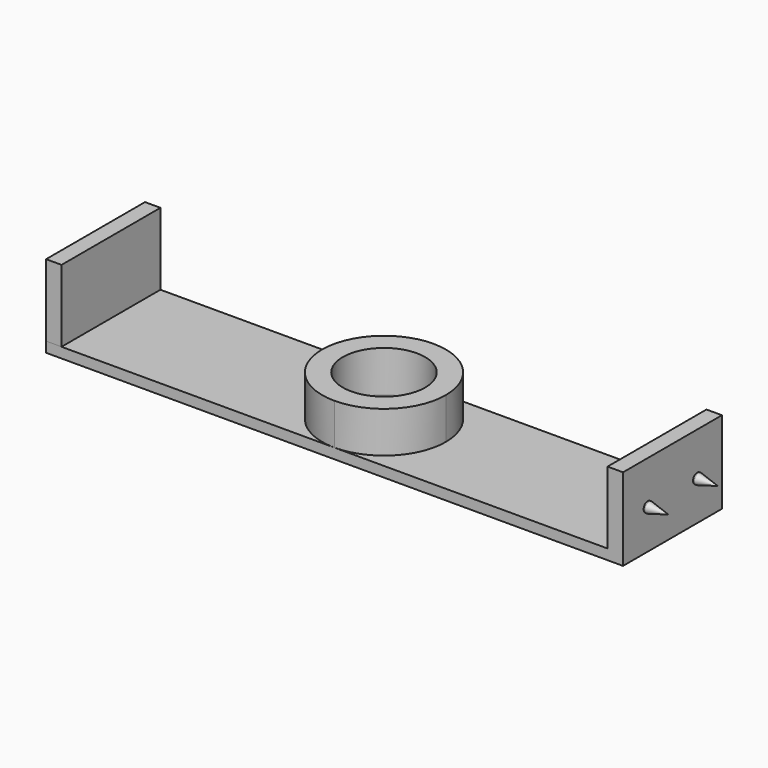
from build123d import *

# Parameters (mm, degrees)
F0_W        = 56
F0_H        = 12
F1_DEPTH    = 1
F2_W        = 12
F2_H        = 12
F2_R        = 4
F3_DEPTH    = 4
F4_DEPTH    = 25
F5_R        = 5.99999
F6_W        = 12
F6_H        = 7
F7_DEPTH    = 1.5
F8_W        = 12
F8_H        = 7
F9_DEPTH    = 1.5
F10_R       = 0.5
F11_DEPTH   = 2
F12_R       = 0.5
F13_DEPTH   = 2
F14_SIZE2   = 1.8660254038
F14_SIZE    = 0.5
F14_2_SIZE2 = 1.8660254038
F14_2_SIZE  = 0.5
F14_3_SIZE2 = 1.8660254038
F14_3_SIZE  = 0.5
F14_4_SIZE2 = 1.8660254038
F14_4_SIZE  = 0.5


# Not quite as in the source:
# - a fillet or chamfer is up to 0.001 mm smaller than in the source, because OpenCascade refuses the exact size


with BuildPart() as f1:
    # F0 (on Top) → F1 (new body)
    with BuildSketch(Plane.XY):
        Rectangle(F0_W, F0_H)
    extrude(amount=F1_DEPTH)

    # F2 (on face) → F3 (join)
    with BuildSketch(Plane.XY.offset(1)):
        Rectangle(F2_W, F2_H)
        Circle(F2_R, mode=Mode.SUBTRACT)
    extrude(amount=F3_DEPTH)

    # F4 (cut): a face of the model
    f4_faces = [f1.faces().sort_by_distance(p)[0] for p in [
        (0, 0, 1),
    ]]
    extrude(f4_faces, amount=-F4_DEPTH, mode=Mode.SUBTRACT)

    # F5 (radius 6 in the source; OpenCascade refuses exactly that, so slightly less here)
    f5_edges = [f1.edges().sort_by_distance(p)[0] for p in [
        (6, 6, 3),
        (6, -6, 3),
        (-6, -6, 3),
        (-6, 6, 3),
    ]]
    fillet(f5_edges, radius=F5_R)

    # F6 (on face) → F7 (join)
    with BuildSketch(Plane.YZ.offset(28)):
        with Locations((0, 4.5)):
            Rectangle(F6_W, F6_H)
    extrude(amount=-F7_DEPTH)

    # F10 (on face) → F11 (join)
    with BuildSketch(Plane.YZ.offset(28)):
        with Locations((3, 3.8193718065)):
            Circle(F10_R)
        with Locations((-3, 3.8193718065)):
            Circle(F10_R)
    extrude(amount=F11_DEPTH)

    # F14
    f14_edges = [f1.edges().sort_by_distance(p)[0] for p in [
        (30, 2.5, 3.819372),
    ]]
    f14_side = f1.faces().sort_by_distance((30, 3, 3.819372))[0]
    chamfer(f14_edges, length=F14_SIZE, length2=F14_SIZE2, reference=f14_side)

    # F14#2
    f14_2_edges = [f1.edges().sort_by_distance(p)[0] for p in [
        (30, -3.5, 3.819372),
    ]]
    f14_2_side = f1.faces().sort_by_distance((30, -3, 3.819372))[0]
    chamfer(f14_2_edges, length=F14_2_SIZE, length2=F14_2_SIZE2, reference=f14_2_side)


with BuildPart() as f9:
    # F8 (on face) → F9 (new body)
    with BuildSketch(Plane(origin=(-28, 0, 0), x_dir=(0, -1, 0), z_dir=(-1, 0, 0))):
        with Locations((0, 4.5)):
            Rectangle(F8_W, F8_H)
    extrude(amount=-F9_DEPTH)

    # F12 (on face) → F13 (join)
    with BuildSketch(Plane(origin=(-28, 0, 0), x_dir=(0, -1, 0), z_dir=(-1, 0, 0))):
        with Locations((3, 4.1950419545)):
            Circle(F12_R)
        with Locations((-3, 4.1950419545)):
            Circle(F12_R)
    extrude(amount=F13_DEPTH)

    # F14#3
    f14_3_edges = [f9.edges().sort_by_distance(p)[0] for p in [
        (-30, -2.5, 4.195042),
    ]]
    f14_3_side = f9.faces().sort_by_distance((-30, -3, 4.195042))[0]
    chamfer(f14_3_edges, length=F14_3_SIZE, length2=F14_3_SIZE2, reference=f14_3_side)

    # F14#4
    f14_4_edges = [f9.edges().sort_by_distance(p)[0] for p in [
        (-30, 3.5, 4.195042),
    ]]
    f14_4_side = f9.faces().sort_by_distance((-30, 3, 4.195042))[0]
    chamfer(f14_4_edges, length=F14_4_SIZE, length2=F14_4_SIZE2, reference=f14_4_side)


solid = Compound([f1.part, f9.part])
